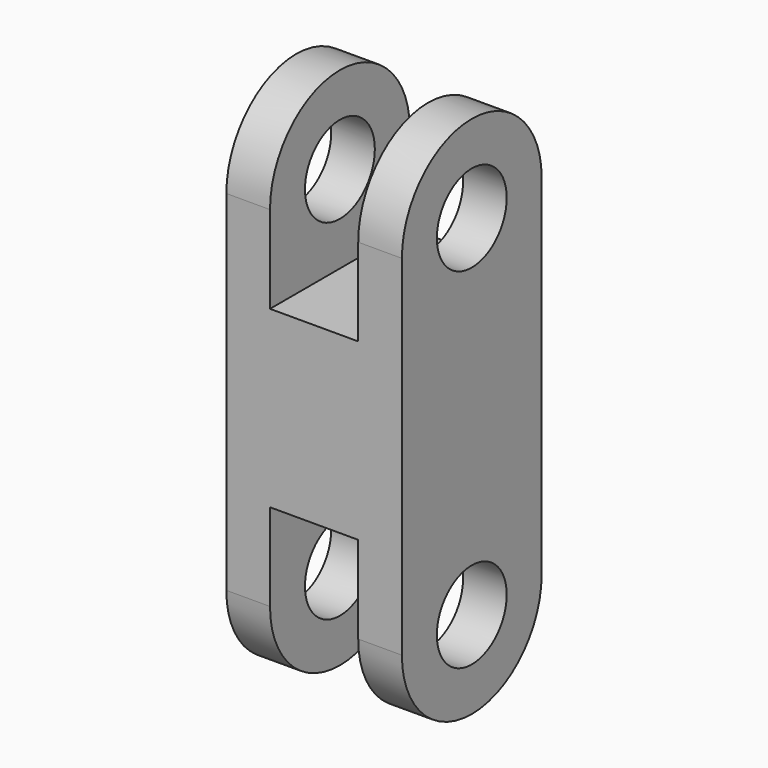
from build123d import *

# Parameters (mm, degrees)
F0_W     = 40
F0_H     = 80
F1_DEPTH = 20.1
F2_R     = 10
F3_DEPTH = 10
F5_W     = 20.2
F5_H     = 40
F6_DEPTH = 40
F7_R     = 10
F8_DEPTH = 40.2
F9_R     = 19.99999


# Not quite as in the source:
# - a fillet or chamfer is up to 0.001 mm smaller than in the source, because OpenCascade refuses the exact size


with BuildPart() as f1:
    # F0 (on Right) → F1 (new body)
    with BuildSketch(Plane.YZ):
        Rectangle(F0_W, F0_H)
    extrude(amount=F1_DEPTH)

    # F2 (on face) → F3 (join)
    with BuildSketch(Plane.YZ.offset(20.1)):
        with BuildLine():
            Line((-20, 60), (-20, 40))
            Line((-20, 40), (20, 40))
            Line((20, 40), (20, 60))
            ThreePointArc((20, 60), (0, 80), (-20, 60))
        make_face()
        with Locations((0, 60)):
            Circle(F2_R, mode=Mode.SUBTRACT)
    extrude(amount=-F3_DEPTH)

    # F4: F1 across face


with BuildPart() as f1_1:
    add(f1.part)
    add(f1.part.mirror(Plane(origin=(0, 0, 0), x_dir=(0, 1, 0), z_dir=(-1, 0, 0))))

    # F5 (on face) → F6 (cut, through all)
    with BuildSketch(Plane.XZ.offset(20)):
        with Locations((0, -20)):
            Rectangle(F5_W, F5_H)
    extrude(amount=-F6_DEPTH, mode=Mode.SUBTRACT)

    # F7 (on face) → F8 (cut, through all)
    with BuildSketch(Plane.YZ.offset(20.1)):
        with Locations((0, -20)):
            Circle(F7_R)
    extrude(amount=-F8_DEPTH, mode=Mode.SUBTRACT)

    # F9 (radius 20 in the source; OpenCascade refuses exactly that, so slightly less here)
    f9_edges = [f1_1.edges().sort_by_distance(p)[0] for p in [
        (-15.1, 20, -40),
        (-15.1, -20, -40),
        (15.1, 20, -40),
        (15.1, -20, -40),
    ]]
    fillet(f9_edges, radius=F9_R)


solid = f1_1.part
